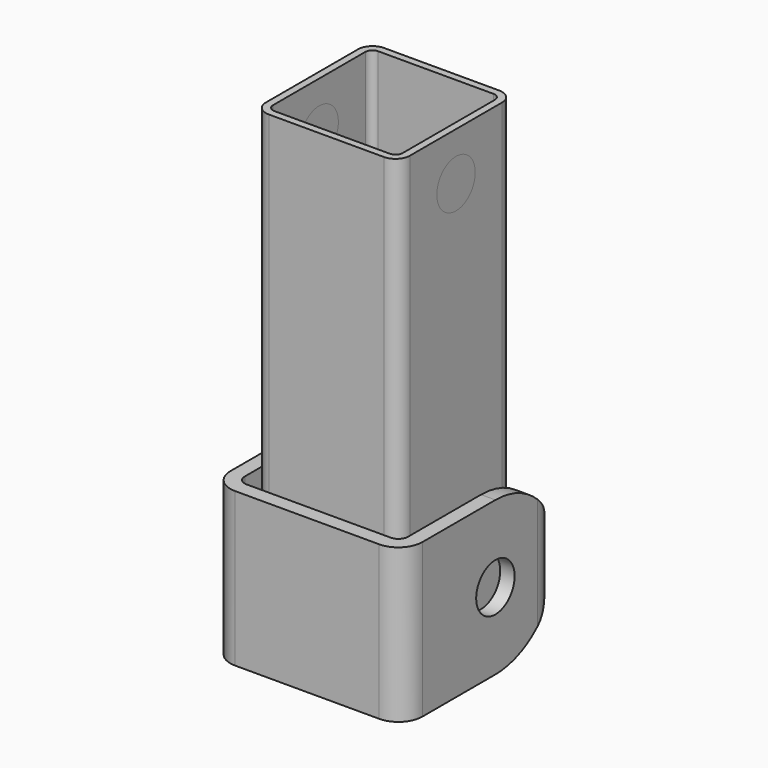
from build123d import *

# Parameters (mm, degrees)
F2_DEPTH  = 100
F3_DEPTH  = 100
F4_R      = 5
F5_DEPTH  = 30.001
F6_DEPTH  = 32
F7_R      = 5
F8_DEPTH  = 40.001
F9_W      = 34
F9_H      = 36.2666666667
F9_W_2    = 30
F9_H_2    = 32
F10_DEPTH = 25
F12_DEPTH = 50


with BuildPart() as f2:
    # F0 (on Top) → F2 (new body)
    with BuildSketch(Plane.XY):
        with BuildLine():
            ThreePointArc((15, 12), (14.1213203436, 14.1213203436), (12, 15))
            Line((12, 15), (-12, 15))
            ThreePointArc((-12, 15), (-14.1213203436, 14.1213203436), (-15, 12))
            Line((-15, 12), (-15, -12))
            ThreePointArc((-15, -12), (-14.1213203436, -14.1213203436), (-12, -15))
            Line((-12, -15), (12, -15))
            ThreePointArc((12, -15), (14.1213203436, -14.1213203436), (15, -12))
            Line((15, -12), (15, 12))
        make_face()
        with BuildLine():
            ThreePointArc((12, 13.5), (13.0606601718, 13.0606601718), (13.5, 12))
            Line((13.5, 12), (13.5, -12))
            ThreePointArc((13.5, -12), (13.0606601718, -13.0606601718), (12, -13.5))
            Line((12, -13.5), (-12, -13.5))
            ThreePointArc((-12, -13.5), (-13.0606601718, -13.0606601718), (-13.5, -12))
            Line((-13.5, -12), (-13.5, 12))
            ThreePointArc((-13.5, 12), (-13.0606601718, 13.0606601718), (-12, 13.5))
            Line((-12, 13.5), (12, 13.5))
        make_face(mode=Mode.SUBTRACT)
    extrude(amount=F2_DEPTH)


with BuildPart() as f3:
    # F0 (on Top) → F3 (new body)
    with BuildSketch(Plane.XY):
        with BuildLine():
            ThreePointArc((15, 12), (14.1213203436, 14.1213203436), (12, 15))
            Line((12, 15), (-12, 15))
            ThreePointArc((-12, 15), (-14.1213203436, 14.1213203436), (-15, 12))
            Line((-15, 12), (-15, -12))
            ThreePointArc((-15, -12), (-14.1213203436, -14.1213203436), (-12, -15))
            Line((-12, -15), (12, -15))
            ThreePointArc((12, -15), (14.1213203436, -14.1213203436), (15, -12))
            Line((15, -12), (15, 12))
        make_face()
        with BuildLine():
            ThreePointArc((12, 13.5), (13.0606601718, 13.0606601718), (13.5, 12))
            Line((13.5, 12), (13.5, -12))
            ThreePointArc((13.5, -12), (13.0606601718, -13.0606601718), (12, -13.5))
            Line((12, -13.5), (-12, -13.5))
            ThreePointArc((-12, -13.5), (-13.0606601718, -13.0606601718), (-13.5, -12))
            Line((-13.5, -12), (-13.5, 12))
            ThreePointArc((-13.5, 12), (-13.0606601718, 13.0606601718), (-12, 13.5))
            Line((-12, 13.5), (12, 13.5))
        make_face(mode=Mode.SUBTRACT)
    extrude(amount=F3_DEPTH)

    # F4 (on face) → F5 (cut, through all)
    with BuildSketch(Plane(origin=(-15, 0, 0), x_dir=(0, -1, 0), z_dir=(-1, 0, 0))):
        with Locations((0, 90)):
            Circle(F4_R)
    extrude(amount=-F5_DEPTH, mode=Mode.SUBTRACT)


with BuildPart() as f6:
    # F1 (on Top) → F6 (new body)
    with BuildSketch(Plane.XY):
        with BuildLine():
            ThreePointArc((20, 15), (18.5355339059, 18.5355339059), (15, 20))
            Line((15, 20), (-15, 20))
            ThreePointArc((-15, 20), (-18.5355339059, 18.5355339059), (-20, 15))
            Line((-20, 15), (-20, -15))
            ThreePointArc((-20, -15), (-18.5355339059, -18.5355339059), (-15, -20))
            Line((-15, -20), (15, -20))
            ThreePointArc((15, -20), (18.5355339059, -18.5355339059), (20, -15))
            Line((20, -15), (20, 15))
        make_face()
        with BuildLine():
            ThreePointArc((15, 17), (16.4142135624, 16.4142135624), (17, 15))
            Line((17, 15), (17, -15))
            ThreePointArc((17, -15), (16.4142135624, -16.4142135624), (15, -17))
            Line((15, -17), (-15, -17))
            ThreePointArc((-15, -17), (-16.4142135624, -16.4142135624), (-17, -15))
            Line((-17, -15), (-17, 15))
            ThreePointArc((-17, 15), (-16.4142135624, 16.4142135624), (-15, 17))
            Line((-15, 17), (15, 17))
        make_face(mode=Mode.SUBTRACT)
    extrude(amount=F6_DEPTH)

    # F7 (on face) → F8 (cut, through all)
    with BuildSketch(Plane(origin=(-20, 0, 0), x_dir=(0, -1, 0), z_dir=(-1, 0, 0))):
        with Locations((-4, 16)):
            Circle(F7_R)
    extrude(amount=-F8_DEPTH, mode=Mode.SUBTRACT)

    # F9 (on face) → F10 (cut)
    with BuildSketch(Plane(origin=(0, 20, 0), x_dir=(-1, 0, 0), z_dir=(0, 1, 0))):
        with Locations((0, 16)):
            Rectangle(F9_W, F9_H)
        with Locations((0, 16)):
            Rectangle(F9_W_2, F9_H_2, mode=Mode.SUBTRACT)
        with Locations((0, 16)):
            Rectangle(F9_W_2, F9_H_2)
    extrude(amount=-F10_DEPTH, mode=Mode.SUBTRACT)

    # F11 (on face) → F12 (cut, symmetric)
    with BuildSketch(Plane.YZ.offset(-17)):
        with BuildLine():
            Line((19.582575695, 32), (4, 32))
            ThreePointArc((4, 32), (13.9475077419, 28.5318430299), (19.582575695, 19.6308862156))
            Line((19.582575695, 19.6308862156), (19.582575695, 32))
        make_face()
        with BuildLine():
            Line((19.582575695, 0), (19.582575695, 12.3691137844))
            ThreePointArc((19.582575695, 12.3691137844), (13.9475077419, 3.4681569701), (4, 0))
            Line((4, 0), (19.582575695, 0))
        make_face()
    extrude(amount=F12_DEPTH, both=True, mode=Mode.SUBTRACT)


solid = Compound([f2.part, f3.part, f6.part])
